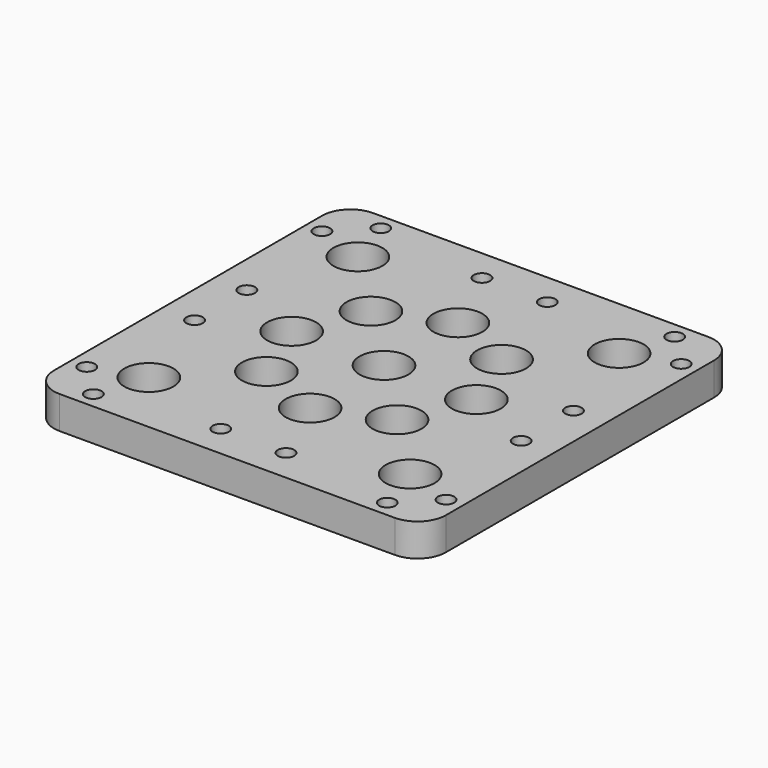
from build123d import *

# Parameters (mm, degrees)
F0_W     = 76.2
F0_H     = 76.2
F0_R     = 1.5875
F0_R_2   = 4.7625
F1_DEPTH = 6.35
F2_R     = 5.5188922036


# Not quite as in the source:
# - a length typed as a fraction of an inch, garbled in the dataset ("3 / 203.2 mm" for 3/8 in), is restored


with BuildPart() as f1:
    # F0 (on Top) → F1 (new body)
    with BuildSketch(Plane.XY):
        Rectangle(F0_W, F0_H)
        with Locations((-28.575, -34.925)):
            Circle(F0_R, mode=Mode.SUBTRACT)
        with Locations((-34.925, -28.575)):
            Circle(F0_R, mode=Mode.SUBTRACT)
        with Locations((-25.4, -25.4)):
            Circle(F0_R_2, mode=Mode.SUBTRACT)
        with Locations((-6.35, -31.75)):
            Circle(F0_R, mode=Mode.SUBTRACT)
        with Locations((-31.75, -6.35)):
            Circle(F0_R, mode=Mode.SUBTRACT)
        with Locations((-12.7, -12.7)):
            Circle(F0_R_2, mode=Mode.SUBTRACT)
        with Locations((6.35, -31.75)):
            Circle(F0_R, mode=Mode.SUBTRACT)
        with Locations((28.575, -34.925)):
            Circle(F0_R, mode=Mode.SUBTRACT)
        with Locations((25.4, -25.4)):
            Circle(F0_R_2, mode=Mode.SUBTRACT)
        with Locations((34.925, -28.575)):
            Circle(F0_R, mode=Mode.SUBTRACT)
        with Locations((0, -17.9605122421)):
            Circle(F0_R_2, mode=Mode.SUBTRACT)
        with Locations((12.7, -12.7)):
            Circle(F0_R_2, mode=Mode.SUBTRACT)
        with Locations((31.75, -6.35)):
            Circle(F0_R, mode=Mode.SUBTRACT)
        with Locations((-31.75, 6.35)):
            Circle(F0_R, mode=Mode.SUBTRACT)
        with Locations((-17.9605122421, 0)):
            Circle(F0_R_2, mode=Mode.SUBTRACT)
        with Locations((-12.7, 12.7)):
            Circle(F0_R_2, mode=Mode.SUBTRACT)
        with Locations((-25.4, 25.4)):
            Circle(F0_R_2, mode=Mode.SUBTRACT)
        with Locations((-34.925, 28.575)):
            Circle(F0_R, mode=Mode.SUBTRACT)
        with Locations((-28.575, 34.925)):
            Circle(F0_R, mode=Mode.SUBTRACT)
        with Locations((-6.35, 31.75)):
            Circle(F0_R, mode=Mode.SUBTRACT)
        Circle(F0_R_2, mode=Mode.SUBTRACT)
        with Locations((17.9605122421, 0)):
            Circle(F0_R_2, mode=Mode.SUBTRACT)
        with Locations((0, 17.9605122421)):
            Circle(F0_R_2, mode=Mode.SUBTRACT)
        with Locations((12.7, 12.7)):
            Circle(F0_R_2, mode=Mode.SUBTRACT)
        with Locations((31.75, 6.35)):
            Circle(F0_R, mode=Mode.SUBTRACT)
        with Locations((6.35, 31.75)):
            Circle(F0_R, mode=Mode.SUBTRACT)
        with Locations((25.4, 25.4)):
            Circle(F0_R_2, mode=Mode.SUBTRACT)
        with Locations((34.925, 28.575)):
            Circle(F0_R, mode=Mode.SUBTRACT)
        with Locations((28.575, 34.925)):
            Circle(F0_R, mode=Mode.SUBTRACT)
    extrude(amount=F1_DEPTH)

    # F2
    f2_edges = [f1.edges().sort_by_distance(p)[0] for p in [
        (-38.1, 38.1, 3.175),
        (-38.1, -38.1, 3.175),
        (38.1, -38.1, 3.175),
        (38.1, 38.1, 3.175),
    ]]
    fillet(f2_edges, radius=F2_R)


solid = f1.part
